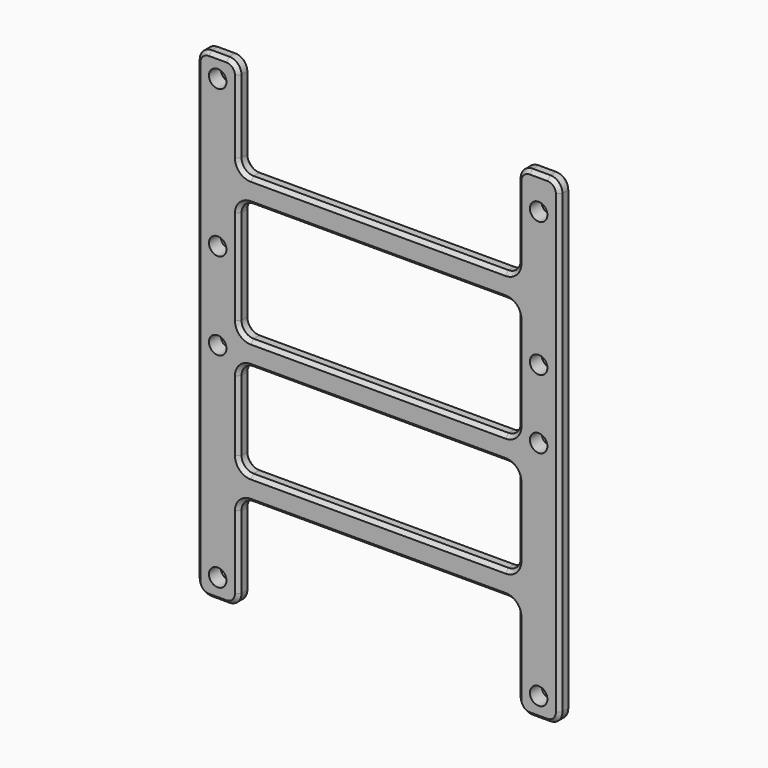
from build123d import *

# Parameters (mm, degrees)
F0_W     = 0.0285906434
F0_H     = 5
F0_W_2   = 28.72
F0_R     = 1.8
F0_W_3   = 57.44
F1_DEPTH = 3
F2_R     = 2.5
F3_SIZE  = 0.75


# Not quite as in the source:
# - a feature names something its author has since deleted; it is built from what else it names


with BuildPart() as f1:
    # F0 (on Front) → F1 (new body)
    with BuildSketch(Plane.XZ):
        with Locations((-28.7342953217, 18.525)):
            Rectangle(F0_W, F0_H)
        with Locations((28.7342953217, 18.525)):
            Rectangle(F0_W, F0_H)
        with Locations((-14.36, 18.525)):
            Rectangle(F0_W_2, F0_H)
        with Locations((14.36, 18.525)):
            Rectangle(F0_W_2, F0_H)
        with Locations((14.36, 42.9671912789)):
            Rectangle(F0_W_2, F0_H)
        Polygon((28.72, 94.9421003461), (28.72, 74.9421003461), (28.72, 69.9421003461), (28.72, 45.4671912789), (28.72, 40.4671912789), (28.72, 21.025), (28.7485906434, 21.025), (28.7485906434, 16.025), (28.72, 16.025), (28.72, -3.975), (37.32, -3.975), (37.32, 94.9421003461), align=None)
        with Locations((33.02, 0.325)):
            Circle(F0_R, mode=Mode.SUBTRACT)
        with Locations((33.02, 46.1421912789)):
            Circle(F0_R, mode=Mode.SUBTRACT)
        with Locations((33.02, 60.325)):
            Circle(F0_R, mode=Mode.SUBTRACT)
        with Locations((33.02, 88.0521912789)):
            Circle(F0_R, mode=Mode.SUBTRACT)
        with Locations((-14.36, 42.9671912789)):
            Rectangle(F0_W_2, F0_H)
        Polygon((-28.72, 94.9421003461), (-37.32, 94.9421003461), (-37.32, -3.975), (-28.72, -3.975), (-28.72, 16.025), (-28.7485906434, 16.025), (-28.7485906434, 21.025), (-28.72, 21.025), (-28.72, 40.4671912789), (-28.72, 45.4671912789), (-28.72, 69.9421003461), (-28.72, 74.9421003461), align=None)
        with Locations((-33.02, 0.325)):
            Circle(F0_R, mode=Mode.SUBTRACT)
        with Locations((-33.02, 42.3821003461)):
            Circle(F0_R, mode=Mode.SUBTRACT)
        with Locations((-33.02, 60.325)):
            Circle(F0_R, mode=Mode.SUBTRACT)
        with Locations((-33.02, 90.6421003461)):
            Circle(F0_R, mode=Mode.SUBTRACT)
        with Locations((0, 72.4421003461)):
            Rectangle(F0_W_3, F0_H)
    extrude(amount=F1_DEPTH)

    # F2
    f2_edges = [f1.edges().sort_by_distance(p)[0] for p in [
        (-28.72, -1.5, 45.467191),
        (28.72, -1.5, 45.467191),
        (-28.72, -1.5, 40.467191),
        (28.72, -1.5, 40.467191),
        (-28.72, -1.5, 21.025),
        (28.72, -1.5, 21.025),
        (-28.72, -1.5, 16.025),
        (28.72, -1.5, 16.025),
        (28.72, -1.5, -3.975),
        (37.32, -1.5, -3.975),
        (-37.32, -1.5, -3.975),
        (-28.72, -1.5, -3.975),
        (37.32, -1.5, 94.9421),
        (28.72, -1.5, 94.9421),
        (-37.32, -1.5, 94.9421),
        (-28.72, -1.5, 94.9421),
        (-28.72, -1.5, 69.9421),
        (28.72, -1.5, 69.9421),
        (-28.72, -1.5, 74.9421),
        (28.72, -1.5, 74.9421),
    ]]
    fillet(f2_edges, radius=F2_R)

    # F3
    f3_edges = [f1.edges().sort_by_distance(p)[0] for p in [
        (0, 0, 16.025),
        (0, 0, 40.467191),
        (-33.02, -3, 94.9421),
        (0, -3, 40.467191),
        (0, -3, 69.9421),
        (0, 0, 69.9421),
    ]]
    chamfer(f3_edges, length=F3_SIZE)


solid = f1.part
